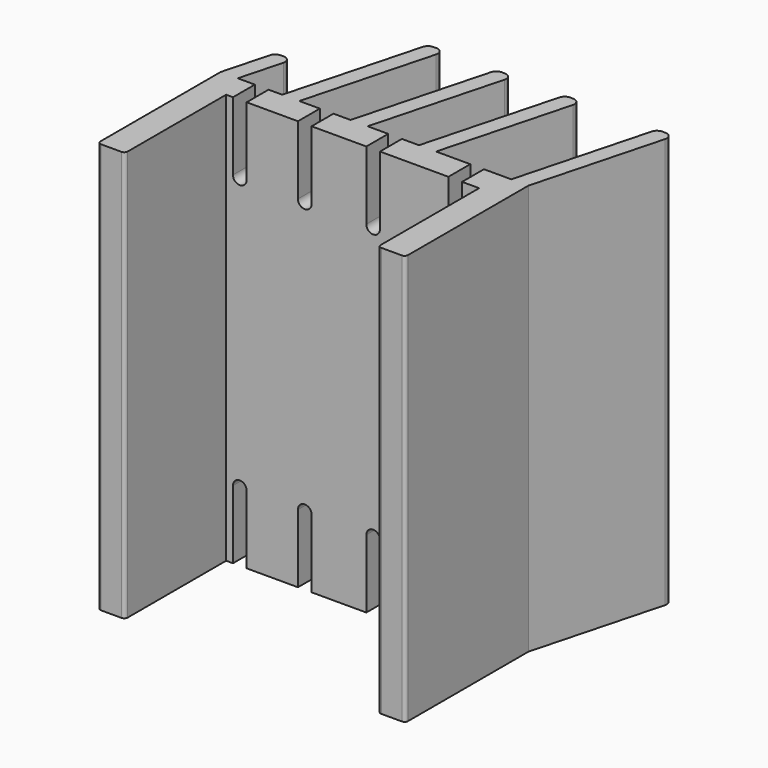
from build123d import *

# Parameters (mm, degrees)
F0_W     = 90
F0_H     = 45
F1_DEPTH = 120
F2_T     = -8
F4_DEPTH = 8
F6_DEPTH = 120
F7_R     = 2
F8_R     = 1


# Not quite as in the source:
# - a feature names something its author has since deleted; it is built from what else it names


with BuildPart() as f1:
    # F0 (on Top) → F1 (new body)
    with BuildSketch(Plane.XY):
        Rectangle(F0_W, F0_H)
    extrude(amount=F1_DEPTH)

    # F2
    f2_openings = [f1.faces().sort_by_distance(p)[0] for p in [
        (0, 0, 120),
        (0, -22.5, 60),
        (0, 0, 0),
    ]]
    offset(amount=F2_T, openings=f2_openings)

    # F3 (on face) → F4 (cut, through all)
    with BuildSketch(Plane(origin=(0, 22.5, 0), x_dir=(-1, 0, 0), z_dir=(0, 1, 0))):
        with BuildLine():
            Line((-32, 20), (-32, 0))
            Line((-32, 0), (-28, 0))
            Line((-28, 0), (-28, 20))
            ThreePointArc((-28, 20), (-30, 22), (-32, 20))
        make_face()
        with BuildLine():
            Line((-8, 20), (-8, 0))
            Line((-8, 0), (-4, 0))
            Line((-4, 0), (-4, 20))
            ThreePointArc((-4, 20), (-6, 22), (-8, 20))
        make_face()
        with BuildLine():
            Line((12, 20), (12, 0))
            Line((12, 0), (16, 0))
            Line((16, 0), (16, 20))
            ThreePointArc((16, 20), (14, 22), (12, 20))
        make_face()
        with BuildLine():
            Line((31, 20), (31, 0))
            Line((31, 0), (35, 0))
            Line((35, 0), (35, 20))
            ThreePointArc((35, 20), (33, 22), (31, 20))
        make_face()
        with BuildLine():
            Line((35, 120), (31, 120))
            Line((31, 120), (31, 100))
            ThreePointArc((31, 100), (33, 98), (35, 100))
            Line((35, 100), (35, 120))
        make_face()
        with BuildLine():
            Line((16, 120), (12, 120))
            Line((12, 120), (12, 100))
            ThreePointArc((12, 100), (14, 98), (16, 100))
            Line((16, 100), (16, 120))
        make_face()
        with BuildLine():
            Line((-4, 120), (-8, 120))
            Line((-8, 120), (-8, 100))
            ThreePointArc((-8, 100), (-6, 98), (-4, 100))
            Line((-4, 100), (-4, 120))
        make_face()
        with BuildLine():
            Line((-28, 120), (-32, 120))
            Line((-32, 120), (-32, 100))
            ThreePointArc((-32, 100), (-30, 98), (-28, 100))
            Line((-28, 100), (-28, 120))
        make_face()
    extrude(amount=-F4_DEPTH, mode=Mode.SUBTRACT)

    # F5 (on face) → F6 (join, through all)
    with BuildSketch(Plane(origin=(0, 0, 0), x_dir=(1, 0, 0), z_dir=(0, 0, -1))):
        Polygon((-40, -22.5), (-45, -22.5), (-41, -37.5), (-36, -37.5), align=None)
        Polygon((-22, -22.5), (-27, -22.5), (-16.3333333333, -62.5), (-11.3333333333, -62.5), align=None)
        Polygon((8.6666666667, -62.5), (-2, -22.5), (-7, -22.5), (3.6666666667, -62.5), align=None)
        Polygon((28.6666666667, -62.5), (18, -22.5), (13, -22.5), (23.6666666667, -62.5), align=None)
        Polygon((45, -22.5), (40, -22.5), (50.6666666667, -62.5), (55.6666666667, -62.5), align=None)
    extrude(amount=-F6_DEPTH)

    # F7
    f7_edges = [f1.edges().sort_by_distance(p)[0] for p in [
        (55.666667, 62.5, 60),
        (50.666667, 62.5, 60),
        (-16.333333, 62.5, 60),
        (3.666667, 62.5, 60),
        (-11.333333, 62.5, 60),
        (-36, 37.5, 60),
        (-41, 37.5, 60),
        (23.666667, 62.5, 60),
        (28.666667, 62.5, 60),
        (8.666667, 62.5, 60),
    ]]
    fillet(f7_edges, radius=F7_R)

    # F8
    f8_edges = [f1.edges().sort_by_distance(p)[0] for p in [
        (-45, -22.5, 60),
        (-37, -22.5, 60),
        (37, -22.5, 60),
        (45, -22.5, 60),
    ]]
    fillet(f8_edges, radius=F8_R)


solid = f1.part
